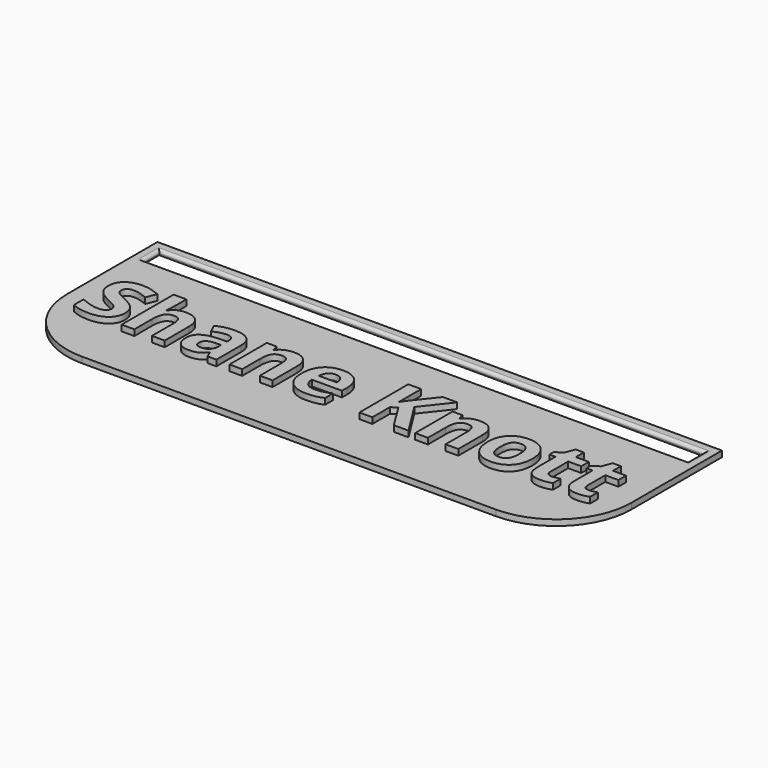
from build123d import *

# Parameters (mm, degrees)
F0_W         = 190.5
F0_H         = 63.5
F1_DEPTH     = 2
F2_W         = 183.896
F2_H         = 7.62
F3_DEPTH     = 25.4
F4_R         = 0.99999
F5_R         = 0.99999
F6_R         = 25.4
F7_TEXT_SIZE = 28.858512338
F8_DEPTH     = 2


# Not quite as in the source:
# - a fillet or chamfer is up to 0.001 mm smaller than in the source, because OpenCascade refuses the exact size
# - Text() gives the source's letters only with a copy of the font that has no kerning and outlines rounded to 1/6400 em; it was checked with that copy


with BuildPart() as f1:
    # F0 (on Top) → F1 (new body)
    with BuildSketch(Plane.XY):
        with Locations((1.791532172, 31.75)):
            Rectangle(F0_W, F0_H)
    extrude(amount=F1_DEPTH)

    # F2 (on face) → F3 (cut)
    with BuildSketch(Plane.XY.offset(2)):
        with Locations((1.791532172, 56.388)):
            Rectangle(F2_W, F2_H)
    extrude(amount=-F3_DEPTH, mode=Mode.SUBTRACT)

    # F4 (radius 1 in the source; OpenCascade refuses exactly that, so slightly less here)
    f4_edges = [f1.edges().sort_by_distance(p)[0] for p in [
        (1.791532, 60.198, 2),
        (1.791532, 60.198, 0),
    ]]
    fillet(f4_edges, radius=F4_R)

    # F5 (radius 1 in the source; OpenCascade refuses exactly that, so slightly less here)
    f5_edges = [f1.edges().sort_by_distance(p)[0] for p in [
        (93.739532, 56.388, 0),
        (93.739532, 56.388, 2),
        (-90.156468, 56.388, 2),
        (-90.156468, 56.388, 0),
    ]]
    fillet(f5_edges, radius=F5_R)

    # F6
    f6_edges = [f1.edges().sort_by_distance(p)[0] for p in [
        (-93.458468, 0, 1),
        (97.041532, 0, 1),
    ]]
    fillet(f6_edges, radius=F6_R)

    # F7 (on face) → F8 (join)
    with BuildSketch(Plane.XY.offset(2)):
        with Locations((-87.108467828, 17.78)):
            Text('Shane Knott', F7_TEXT_SIZE, font='Open Sans', font_style=FontStyle.BOLD, text_align=(TextAlign.LEFT, TextAlign.BOTTOM))
    extrude(amount=F8_DEPTH)


solid = f1.part
